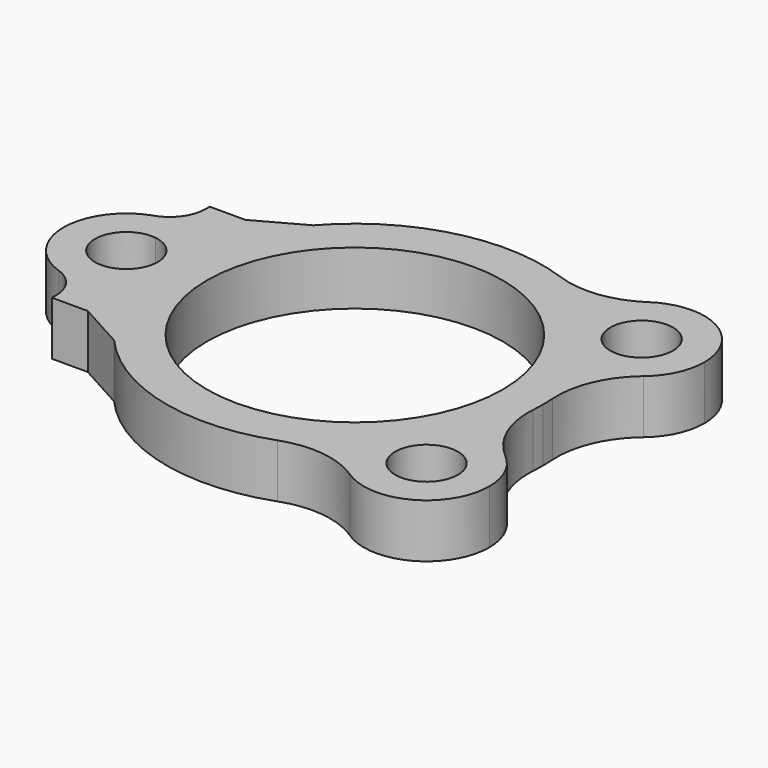
from build123d import *

# Parameters (mm, degrees)
F0_R     = 8.25
F0_R_2   = 1.75
F1_DEPTH = 3
F2_R     = 2
F3_R     = 5


# Not quite as in the source:
# - a feature names something its author has since deleted; it is built from what else it names


with BuildPart() as f1:
    # F0 (on Top) → F1 (new body)
    with BuildSketch(Plane.XY):
        with BuildLine():
            Line((-10.5, -2.6809513237), (-10.5, 0))
            Line((-10.5, 0), (-10.5, 2.6809513237))
            ThreePointArc((-10.5, 2.6809513237), (-11.4360102659, 3.243983813), (-12.5, 3.4910600109))
            Line((-12.5, 3.4910600109), (-12.5, 1.7320508076))
            ThreePointArc((-12.5, 1.7320508076), (-11.4271243445, 1.1456439237), (-11, 0))
            ThreePointArc((-11, 0), (-11.4271243445, -1.1456439237), (-12.5, -1.7320508076))
            Line((-12.5, -1.7320508076), (-12.5, -3.4910600109))
            ThreePointArc((-12.5, -3.4910600109), (-11.4360102659, -3.243983813), (-10.5, -2.6809513237))
        make_face()
        with BuildLine():
            Line((-12.5, 1.7320508076), (-12.5, 3.4910600109))
            ThreePointArc((-12.5, 3.4910600109), (-16.25, 0), (-12.5, -3.4910600109))
            Line((-12.5, -3.4910600109), (-12.5, -1.7320508076))
            ThreePointArc((-12.5, -1.7320508076), (-14.5, 0), (-12.5, 1.7320508076))
        make_face()
        with BuildLine():
            Line((-10.5, 2.6809513237), (-10.5, 5.5))
            Line((-10.5, 5.5), (-12.5, 5.5))
            Line((-12.5, 5.5), (-12.5, 3.4910600109))
            ThreePointArc((-12.5, 3.4910600109), (-11.4360102659, 3.243983813), (-10.5, 2.6809513237))
        make_face()
        with BuildLine():
            ThreePointArc((-10.2181372549, 2.4165411314), (-9.3247712996, 4.8268665001), (-7.8725304742, 6.9478963675))
            Line((-7.8725304742, 6.9478963675), (-10.5, 5.5))
            Line((-10.5, 5.5), (-10.5, 2.6809513237))
            ThreePointArc((-10.5, 2.6809513237), (-10.3554163168, 2.5526396111), (-10.2181372549, 2.4165411314))
        make_face()
        with BuildLine():
            Line((-7.2260237528, 5.7746931281), (-7.8725304742, 6.9478963675))
            ThreePointArc((-7.8725304742, 6.9478963675), (-9.3247712996, 4.8268665001), (-10.2181372549, 2.4165411314))
            ThreePointArc((-10.2181372549, 2.4165411314), (-9.5010371187, 1.301629823), (-9.25, 0))
            ThreePointArc((-9.25, 0), (-8.729353347, 3.0595571809), (-7.2260237528, 5.7746931281))
        make_face()
        with BuildLine():
            ThreePointArc((6.6767394005, 6.401847466), (6.5063300085, 7.2895956499), (6.5689658587, 8.1913788551))
            ThreePointArc((6.5689658587, 8.1913788551), (-0.9007676454, 10.4612913949), (-7.8725304742, 6.9478963675))
            Line((-7.8725304742, 6.9478963675), (-7.2260237528, 5.7746931281))
            ThreePointArc((-7.2260237528, 5.7746931281), (-0.4168440545, 9.2406028502), (6.6767394005, 6.401847466))
        make_face()
        with BuildLine():
            ThreePointArc((9.25, 0), (8.9359851316, 2.3897007611), (8.0152605995, 4.617152534))
            ThreePointArc((8.0152605995, 4.617152534), (7.2, 5.4), (6.6767394005, 6.401847466))
            ThreePointArc((6.6767394005, 6.401847466), (-0.4168440545, 9.2406028502), (-7.2260237528, 5.7746931281))
            ThreePointArc((-7.2260237528, 5.7746931281), (-8.729353347, 3.0595571809), (-9.25, 0))
            ThreePointArc((-9.25, 0), (-8.729353347, -3.0595571809), (-7.2260237528, -5.7746931281))
            ThreePointArc((-7.2260237528, -5.7746931281), (-0.4168440545, -9.2406028502), (6.6767394005, -6.401847466))
            ThreePointArc((6.6767394005, -6.401847466), (7.2, -5.4), (8.0152605995, -4.617152534))
            ThreePointArc((8.0152605995, -4.617152534), (8.9359851316, -2.3897007611), (9.25, 0))
        make_face()
        Circle(F0_R, mode=Mode.SUBTRACT)
        with BuildLine():
            Line((-12.5, -5.5), (-10.5, -5.5))
            Line((-10.5, -5.5), (-10.5, -2.6809513237))
            ThreePointArc((-10.5, -2.6809513237), (-11.4360102659, -3.243983813), (-12.5, -3.4910600109))
            Line((-12.5, -3.4910600109), (-12.5, -5.5))
        make_face()
        with BuildLine():
            Line((-10.5, -5.5), (-7.8725304742, -6.9478963675))
            ThreePointArc((-7.8725304742, -6.9478963675), (-9.3247712996, -4.8268665001), (-10.2181372549, -2.4165411314))
            ThreePointArc((-10.2181372549, -2.4165411314), (-10.3554163168, -2.5526396111), (-10.5, -2.6809513237))
            Line((-10.5, -2.6809513237), (-10.5, -5.5))
        make_face()
        with BuildLine():
            ThreePointArc((-10.5, -2.6809513237), (-10.3554163168, -2.5526396111), (-10.2181372549, -2.4165411314))
            ThreePointArc((-10.2181372549, -2.4165411314), (-10.4292962652, -1.2164618415), (-10.5, 0))
            Line((-10.5, 0), (-10.5, -2.6809513237))
        make_face()
        with BuildLine():
            ThreePointArc((-9.25, 0), (-9.5010371187, 1.301629823), (-10.2181372549, 2.4165411314))
            ThreePointArc((-10.2181372549, 2.4165411314), (-10.4292962652, 1.2164618415), (-10.5, 0))
            ThreePointArc((-10.5, 0), (-10.4292962652, -1.2164618415), (-10.2181372549, -2.4165411314))
            ThreePointArc((-10.2181372549, -2.4165411314), (-9.5010371187, -1.301629823), (-9.25, 0))
        make_face()
        with BuildLine():
            ThreePointArc((-10.2181372549, -2.4165411314), (-9.3247712996, -4.8268665001), (-7.8725304742, -6.9478963675))
            Line((-7.8725304742, -6.9478963675), (-7.2260237528, -5.7746931281))
            ThreePointArc((-7.2260237528, -5.7746931281), (-8.729353347, -3.0595571809), (-9.25, 0))
            ThreePointArc((-9.25, 0), (-9.5010371187, -1.301629823), (-10.2181372549, -2.4165411314))
        make_face()
        with BuildLine():
            ThreePointArc((-10.5, 0), (-10.4292962652, 1.2164618415), (-10.2181372549, 2.4165411314))
            ThreePointArc((-10.2181372549, 2.4165411314), (-10.3554163168, 2.5526396111), (-10.5, 2.6809513237))
            Line((-10.5, 2.6809513237), (-10.5, 0))
        make_face()
        with BuildLine():
            ThreePointArc((-7.8725304742, -6.9478963675), (-0.9007676454, -10.4612913949), (6.5689658587, -8.1913788551))
            ThreePointArc((6.5689658587, -8.1913788551), (6.5063300085, -7.2895956499), (6.6767394005, -6.401847466))
            ThreePointArc((6.6767394005, -6.401847466), (-0.4168440545, -9.2406028502), (-7.2260237528, -5.7746931281))
            Line((-7.2260237528, -5.7746931281), (-7.8725304742, -6.9478963675))
        make_face()
        with BuildLine():
            ThreePointArc((6.5689658587, -8.1913788551), (8.4, -6.3), (9.7030341413, -4.0126211449))
            ThreePointArc((9.7030341413, -4.0126211449), (8.8197842263, -4.2049900262), (8.0152605995, -4.617152534))
            ThreePointArc((8.0152605995, -4.617152534), (7.4, -5.55), (6.6767394005, -6.401847466))
            ThreePointArc((6.6767394005, -6.401847466), (6.5063300085, -7.2895956499), (6.5689658587, -8.1913788551))
        make_face()
        with BuildLine():
            ThreePointArc((13.5, -7.5), (12.3675535363, -4.9222703298), (9.7030341413, -4.0126211449))
            ThreePointArc((9.7030341413, -4.0126211449), (8.4, -6.3), (6.5689658587, -8.1913788551))
            ThreePointArc((6.5689658587, -8.1913788551), (10.3474050269, -10.982715858), (13.5, -7.5))
        make_face()
        with Locations((10, -7.5)):
            Circle(F0_R_2, mode=Mode.SUBTRACT)
        with BuildLine():
            ThreePointArc((6.6767394005, -6.401847466), (7.4, -5.55), (8.0152605995, -4.617152534))
            ThreePointArc((8.0152605995, -4.617152534), (7.2, -5.4), (6.6767394005, -6.401847466))
        make_face()
        with BuildLine():
            ThreePointArc((9.7030341413, -4.0126211449), (10.2988314503, -2.0455001242), (10.5, 0))
            ThreePointArc((10.5, 0), (10.2988314503, 2.0455001242), (9.7030341413, 4.0126211449))
            ThreePointArc((9.7030341413, 4.0126211449), (8.8197842263, 4.2049900262), (8.0152605995, 4.617152534))
            ThreePointArc((8.0152605995, 4.617152534), (8.9359851316, 2.3897007611), (9.25, 0))
            ThreePointArc((9.25, 0), (8.9359851316, -2.3897007611), (8.0152605995, -4.617152534))
            ThreePointArc((8.0152605995, -4.617152534), (8.8197842263, -4.2049900262), (9.7030341413, -4.0126211449))
        make_face()
        with BuildLine():
            ThreePointArc((6.6767394005, 6.401847466), (7.2, 5.4), (8.0152605995, 4.617152534))
            ThreePointArc((8.0152605995, 4.617152534), (7.4, 5.55), (6.6767394005, 6.401847466))
        make_face()
        with BuildLine():
            ThreePointArc((8.0152605995, 4.617152534), (8.8197842263, 4.2049900262), (9.7030341413, 4.0126211449))
            ThreePointArc((9.7030341413, 4.0126211449), (8.4, 6.3), (6.5689658587, 8.1913788551))
            ThreePointArc((6.5689658587, 8.1913788551), (6.5063300085, 7.2895956499), (6.6767394005, 6.401847466))
            ThreePointArc((6.6767394005, 6.401847466), (7.4, 5.55), (8.0152605995, 4.617152534))
        make_face()
        with BuildLine():
            ThreePointArc((6.5689658587, 8.1913788551), (8.4, 6.3), (9.7030341413, 4.0126211449))
            ThreePointArc((9.7030341413, 4.0126211449), (12.3675535363, 4.9222703298), (13.5, 7.5))
            ThreePointArc((13.5, 7.5), (10.3474050269, 10.982715858), (6.5689658587, 8.1913788551))
        make_face()
        with Locations((10, 7.5)):
            Circle(F0_R_2, mode=Mode.SUBTRACT)
    extrude(amount=F1_DEPTH)

    # F2
    f2_edges = [f1.edges().sort_by_distance(p)[0] for p in [
        (-12.5, -3.49106, 1.5),
        (-12.5, 3.49106, 1.5),
    ]]
    fillet(f2_edges, radius=F2_R)

    # F3
    f3_edges = [f1.edges().sort_by_distance(p)[0] for p in [
        (6.568966, -8.191379, 1.5),
        (9.703034, -4.012621, 1.5),
        (9.703034, 4.012621, 1.5),
        (6.568966, 8.191379, 1.5),
    ]]
    fillet(f3_edges, radius=F3_R)


solid = f1.part
